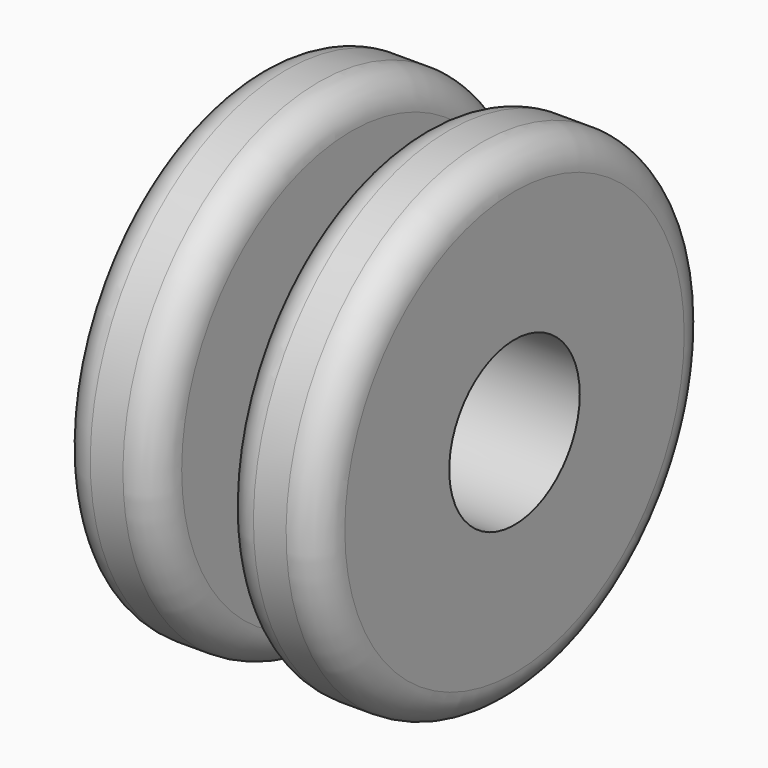
from build123d import *

# Parameters (mm, degrees)
F2_R     = 1.26999
F3_R     = 3.175
F4_DEPTH = 25.4


# Not quite as in the source:
# - a fillet or chamfer is up to 0.001 mm smaller than in the source, because OpenCascade refuses the exact size


with BuildPart() as f1:
    # F0 (on Front) → F1 (revolve)
    with BuildSketch(Plane.XZ):
        Polygon((0, 9.525), (0, 0), (10.16, 0), (10.16, 9.525), (6.35, 9.525), (6.35, 3.175), (3.81, 3.175), (3.81, 9.525), align=None)
    revolve(axis=Axis((5.08, 0, 0), (1, 0, 0)))

    # F2 (radius 1.27 in the source; OpenCascade refuses exactly that, so slightly less here)
    f2_edges = [f1.edges().sort_by_distance(p)[0] for p in [
        (10.16, 0, -9.525),
        (6.35, 0, -9.525),
        (3.81, 0, -9.525),
        (0, 0, -9.525),
        (3.81, 0, -3.175),
        (6.35, 0, -3.175),
    ]]
    fillet(f2_edges, radius=F2_R)

    # F3 (on face) → F4 (cut)
    with BuildSketch(Plane.YZ.offset(10.16)):
        Circle(F3_R)
    extrude(amount=-F4_DEPTH, mode=Mode.SUBTRACT)


solid = f1.part
